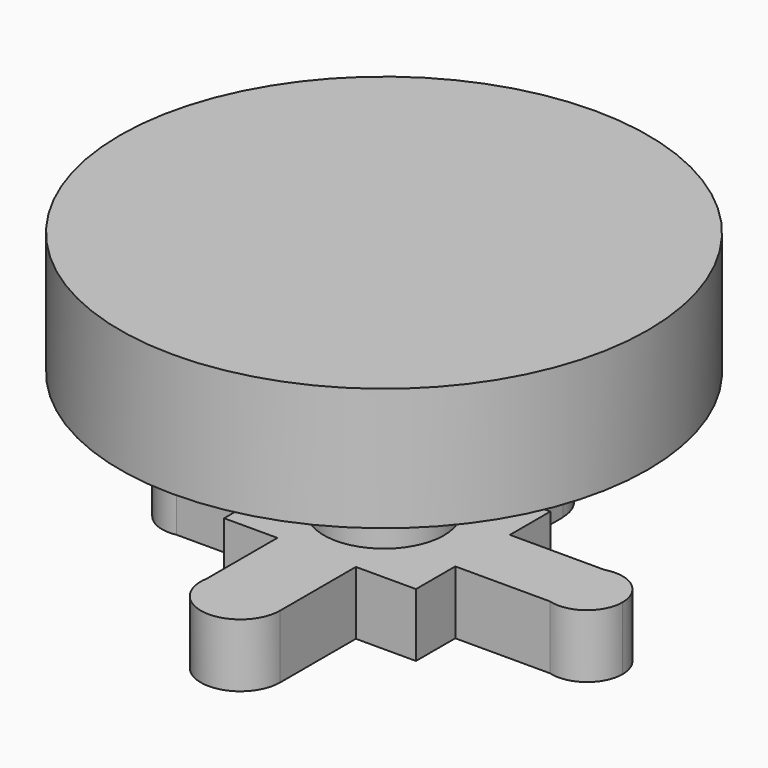
from build123d import *

# Parameters (mm, degrees)
F2_W     = 17.3420682549
F2_H     = 35.8665511012
F4_R     = 17.3420682549
F5_DEPTH = 18.288


# Not quite as in the source:
# - the program builds the solid bodies; features that only make, move or delete a surface that nothing else refers to are left out


with BuildPart() as f1:
    # F0 (on Front) → F1 (revolve)
    with BuildSketch(Plane.XZ):
        with BuildLine():
            Line((0, 0), (35.2114337626, 0))
            ThreePointArc((35.2114337626, 0), (24.8982435888, 24.8982435888), (0, 35.2114337626))
            Line((0, 35.2114337626), (0, 0))
        make_face()
        with BuildLine():
            ThreePointArc((0, 35.2114337626), (24.8982435888, 24.8982435888), (35.2114337626, 0))
            Line((35.2114337626, 0), (76.2656927109, 0))
            Line((76.2656927109, 0), (76.2656927109, 35.4724153876))
            Line((76.2656927109, 35.4724153876), (0, 35.4724153876))
            Line((0, 35.4724153876), (0, 35.2114337626))
        make_face()
    revolve(axis=Axis((0, 0, 17.7362076938), (0, 0, 1)))

    # F2 (on Front) → F3 (revolve)
    with BuildSketch(Plane.XZ):
        with Locations((8.6710341275, -17.9332755506)):
            Rectangle(F2_W, F2_H)
    revolve(axis=Axis((0, 0, -17.9332755506), (0, 0, -1)))


with BuildPart() as f5:
    # F4 (on face) → F5 (new body)
    with BuildSketch(Plane(origin=(0, 0, -35.8665511012), x_dir=(1, 0, 0), z_dir=(0, 0, -1))):
        with BuildLine():
            Line((56.1504008339, 10.256420821), (28.7968739867, 10.256420821))
            Line((28.7968739867, 10.256420821), (28.7968739867, -9.467465803))
            Line((28.7968739867, -9.467465803), (56.1504008339, -9.467465803))
            ThreePointArc((56.1504008339, -9.467465803), (48.7161076265, 0.394477509), (56.1504008339, 10.256420821))
        make_face()
        Polygon((28.7968739867, 10.256420821), (28.7968739867, 24.4576204568), (11.4398542792, 24.4576204568), (-11.242615059, 24.4576204568), (-26.6272462904, 24.4576204568), (-26.6272462904, 10.0591816008), (-26.6272462904, -10.256420821), (-26.6272462904, -24.0631420165), (-12.623286806, -24.0631420165), (10.8481375501, -24.0631420165), (28.7968739867, -24.0631420165), (28.7968739867, -9.467465803), align=None)
        Circle(F4_R, mode=Mode.SUBTRACT)
        with BuildLine():
            Line((10.8481375501, -51.0848648846), (10.8481375501, -24.0631420165))
            Line((10.8481375501, -24.0631420165), (-12.623286806, -24.0631420165))
            Line((-12.623286806, -24.0631420165), (-12.623286806, -51.0848648846))
            Line((-12.623286806, -51.0848648846), (-12.5334393836, -51.0848648846))
            ThreePointArc((-12.5334393836, -51.0848648846), (-0.887574628, -39.4390001291), (10.7582901276, -51.0848648846))
            Line((10.7582901276, -51.0848648846), (10.8481375501, -51.0848648846))
        make_face()
        with BuildLine():
            Line((-26.6272462904, -10.256420821), (-26.6272462904, 10.0591816008))
            Line((-26.6272462904, 10.0591816008), (-51.8444488937, 10.0591816008))
            ThreePointArc((-51.8444488937, 10.0591816008), (-45.9176178455, 6.5062777185), (-43.5897856951, 0))
            ThreePointArc((-43.5897856951, 0), (-46.5938218028, -7.2523847132), (-53.846206516, -10.256420821))
            Line((-53.846206516, -10.256420821), (-26.6272462904, -10.256420821))
        make_face()
        with BuildLine():
            Line((-11.242615059, 24.4576204568), (11.4398542792, 24.4576204568))
            Line((11.4398542792, 24.4576204568), (11.4398542792, 51.8738217652))
            Line((11.4398542792, 51.8738217652), (11.4143216161, 51.8738217652))
            ThreePointArc((11.4143216161, 51.8738217652), (0.9899277412, 40.502507812), (-11.242615059, 49.9014261179))
            Line((-11.242615059, 49.9014261179), (-11.242615059, 24.4576204568))
        make_face()
        with BuildLine():
            ThreePointArc((69.2327374024, 0.394477509), (65.1495063475, 8.5860197322), (56.1504008339, 10.256420821))
            Line((56.1504008339, 10.256420821), (58.9744225144, 10.256420821))
            Line((58.9744225144, 10.256420821), (58.9744225144, -9.467465803))
            Line((58.9744225144, -9.467465803), (56.1504008339, -9.467465803))
            ThreePointArc((56.1504008339, -9.467465803), (65.1495063475, -7.7970647143), (69.2327374024, 0.394477509))
        make_face()
        with BuildLine():
            ThreePointArc((-12.5334393836, -51.0848648846), (-0.887574628, -62.7307296402), (10.7582901276, -51.0848648846))
            Line((10.7582901276, -51.0848648846), (-12.5334393836, -51.0848648846))
        make_face()
        with BuildLine():
            Line((-53.846206516, 10.0591816008), (-51.8444488937, 10.0591816008))
            ThreePointArc((-51.8444488937, 10.0591816008), (-64.0531984252, 1.0057257191), (-53.846206516, -10.256420821))
            Line((-53.846206516, -10.256420821), (-53.846206516, 10.0591816008))
        make_face()
        with BuildLine():
            Line((-12.5334393836, -51.0848648846), (10.7582901276, -51.0848648846))
            ThreePointArc((10.7582901276, -51.0848648846), (-0.887574628, -39.4390001291), (-12.5334393836, -51.0848648846))
        make_face()
        with BuildLine():
            Line((58.9744225144, 10.256420821), (56.1504008339, 10.256420821))
            ThreePointArc((56.1504008339, 10.256420821), (48.7161076265, 0.394477509), (56.1504008339, -9.467465803))
            Line((56.1504008339, -9.467465803), (58.9744225144, -9.467465803))
            Line((58.9744225144, -9.467465803), (58.9744225144, 10.256420821))
        make_face()
        with BuildLine():
            Line((-11.242615059, 51.8738217652), (-11.242615059, 49.9014261179))
            ThreePointArc((-11.242615059, 49.9014261179), (0.9899277412, 40.502507812), (11.4143216161, 51.8738217652))
            Line((11.4143216161, 51.8738217652), (-11.242615059, 51.8738217652))
        make_face()
        with BuildLine():
            ThreePointArc((11.4143216161, 51.8738217652), (-0.9899277412, 63.2451357184), (-11.242615059, 49.9014261179))
            Line((-11.242615059, 49.9014261179), (-11.242615059, 51.8738217652))
            Line((-11.242615059, 51.8738217652), (11.4143216161, 51.8738217652))
        make_face()
        with BuildLine():
            ThreePointArc((-43.5897856951, 0), (-45.9176178455, 6.5062777185), (-51.8444488937, 10.0591816008))
            Line((-51.8444488937, 10.0591816008), (-53.846206516, 10.0591816008))
            Line((-53.846206516, 10.0591816008), (-53.846206516, -10.256420821))
            ThreePointArc((-53.846206516, -10.256420821), (-46.5938218028, -7.2523847132), (-43.5897856951, 0))
        make_face()
    extrude(amount=F5_DEPTH)


solid = Compound([f1.part, f5.part])
